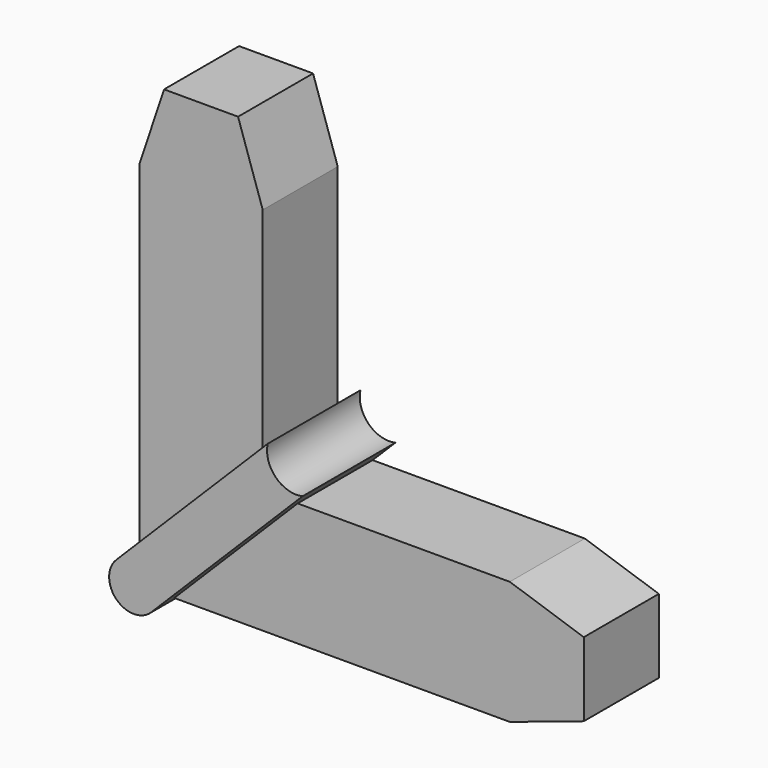
from build123d import *

# Parameters (mm, degrees)
F1_DEPTH   = 11.938
F2_DEPTH   = 9.652
F3_SIZE2   = 2.54
F3_SIZE    = 7.62
F3_2_SIZE2 = 2.54
F3_2_SIZE  = 7.62
F3_3_SIZE2 = 2.54
F3_3_SIZE  = 7.62
F4_SIZE2   = 7.62
F4_SIZE    = 2.54
F5_R       = 2.53999
F6_R       = 3.0383713325
F7_DEPTH   = 25.4


# Not quite as in the source:
# - a fillet or chamfer is up to 0.001 mm smaller than in the source, because OpenCascade refuses the exact size


with BuildPart() as f1:
    # F0 (on Front) → F1 (new body)
    with BuildSketch(Plane.XZ):
        Polygon((-6.8888153673, -10.4809178157), (-4.5539487758, -8.1460512242), (8.1460512242, 4.5539487758), (10.4809178157, 6.8888153673), (6.8888153673, 10.4809178157), (4.5539487758, 8.1460512242), (-8.1460512242, -4.5539487758), (-10.4809178157, -6.8888153673), align=None)
    extrude(amount=F1_DEPTH)

    # F0 (on Front) → F2 (join)
    with BuildSketch(Plane.XZ):
        Polygon((-8.1460512242, 37.6100512242), (-8.1460512242, -4.5539487758), (4.5539487758, 8.1460512242), (4.5539487758, 37.6100512242), (0, 37.6100512242), align=None)
        Polygon((8.1460512242, 4.5539487758), (-4.5539487758, -8.1460512242), (37.6100512242, -8.1460512242), (37.6100512242, 0), (37.6100512242, 4.5539487758), align=None)
    extrude(amount=F2_DEPTH)

    # F3
    f3_edges = [f1.edges().sort_by_distance(p)[0] for p in [
        (-8.146051, -4.826, 37.610051),
    ]]
    f3_side = f1.faces().sort_by_distance((-8.146051, -4.826, 16.528051))[0]
    chamfer(f3_edges, length=F3_SIZE, length2=F3_SIZE2, reference=f3_side)

    # F3#2
    f3_2_edges = [f1.edges().sort_by_distance(p)[0] for p in [
        (4.553949, -4.826, 37.610051),
    ]]
    f3_2_side = f1.faces().sort_by_distance((4.553949, -4.826, 22.878051))[0]
    chamfer(f3_2_edges, length=F3_2_SIZE, length2=F3_2_SIZE2, reference=f3_2_side)

    # F3#3
    f3_3_edges = [f1.edges().sort_by_distance(p)[0] for p in [
        (37.610051, -4.826, 4.553949),
    ]]
    f3_3_side = f1.faces().sort_by_distance((22.878051, -4.826, 4.553949))[0]
    chamfer(f3_3_edges, length=F3_3_SIZE, length2=F3_3_SIZE2, reference=f3_3_side)

    # F4
    f4_edges = [f1.edges().sort_by_distance(p)[0] for p in [
        (37.610051, -4.826, -8.146051),
    ]]
    f4_side = f1.faces().sort_by_distance((37.610051, -4.826, -3.066051))[0]
    chamfer(f4_edges, length=F4_SIZE, length2=F4_SIZE2, reference=f4_side)

    # F5 (radius 2.54 in the source; OpenCascade refuses exactly that, so slightly less here)
    f5_edges = [f1.edges().sort_by_distance(p)[0] for p in [
        (-10.480918, -5.969, -6.888815),
        (-6.888815, -5.969, -10.480918),
    ]]
    fillet(f5_edges, radius=F5_R)

    # F6 (on face) → F7 (cut)
    with BuildSketch(Plane.XZ.offset(11.938)):
        with Locations((9.8638704833, 9.8638704833)):
            Circle(F6_R)
    extrude(amount=-F7_DEPTH, mode=Mode.SUBTRACT)


solid = f1.part
